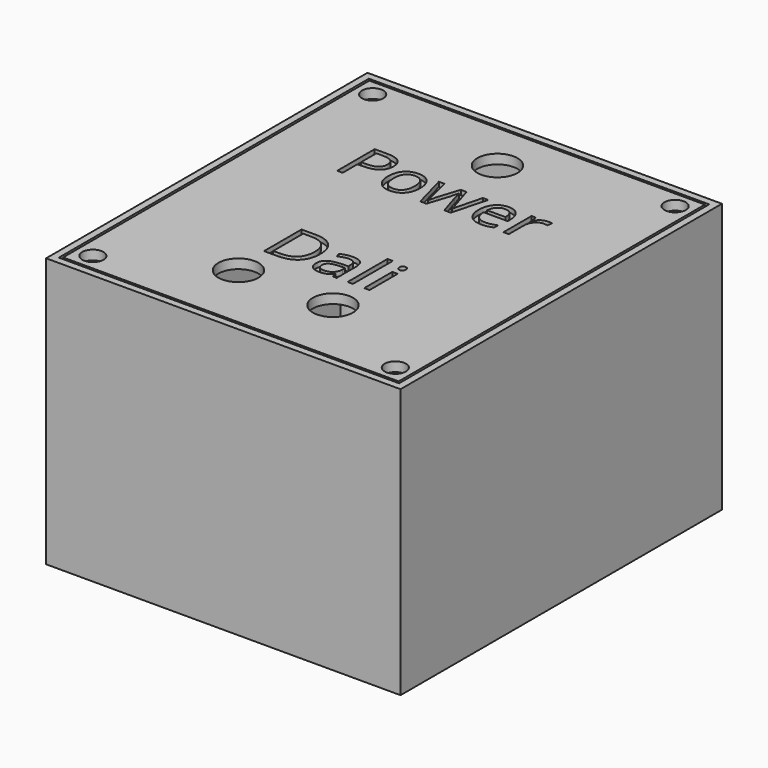
from build123d import *

# Parameters (mm, degrees)
F0_W          = 75
F0_H          = 85
F0_W_2        = 53
F0_H_2        = 63
F0_R          = 4
F1_DEPTH      = 2
F2_DEPTH      = 57
F3_DEPTH      = 9
F4_W          = 72
F4_H          = 82
F5_DEPTH      = 2
F6_D          = 3.2
F8_D          = 3.2
F8_DEPTH      = 12
F8_TIP        = 0.9613769904
F9_W          = 71
F9_H          = 81
F10_DEPTH     = 2
F11_D         = 4.5
F11_DEPTH     = 12
F11_TIP       = 1.3519363928
F13_D         = 8.5
F12_TEXT_SIZE = 13.8888888889
F14_DEPTH     = 1


# Not quite as in the source:
# - Text() gives the source's letters only with a copy of the font that has no kerning and outlines rounded to 1/6400 em; it was checked with that copy


with BuildPart() as f1:
    # F0 (on Top) → F1 (new body)
    with BuildSketch(Plane.XY):
        Rectangle(F0_W, F0_H)
        with BuildLine():
            ThreePointArc((-34, 31), (-28.3431457505, 33.3431457505), (-26, 39))
            Line((-26, 39), (26, 39))
            ThreePointArc((26, 39), (28.3431457505, 33.3431457505), (34, 31))
            Line((34, 31), (34, -31))
            ThreePointArc((34, -31), (28.3431457505, -33.3431457505), (26, -39))
            Line((26, -39), (-26, -39))
            ThreePointArc((-26, -39), (-28.3431457505, -33.3431457505), (-34, -31))
            Line((-34, -31), (-34, 31))
        make_face(mode=Mode.SUBTRACT)
        with BuildLine():
            Line((26, 39), (-26, 39))
            ThreePointArc((-26, 39), (-28.3431457505, 33.3431457505), (-34, 31))
            Line((-34, 31), (-34, -31))
            ThreePointArc((-34, -31), (-28.3431457505, -33.3431457505), (-26, -39))
            Line((-26, -39), (26, -39))
            ThreePointArc((26, -39), (28.3431457505, -33.3431457505), (34, -31))
            Line((34, -31), (34, 31))
            ThreePointArc((34, 31), (28.3431457505, 33.3431457505), (26, 39))
        make_face()
        Rectangle(F0_W_2, F0_H_2, mode=Mode.SUBTRACT)
        Rectangle(F0_W_2, F0_H_2)
        with Locations((-21.5, -26.5)):
            Circle(F0_R, mode=Mode.SUBTRACT)
        with Locations((21.5, -26.5)):
            Circle(F0_R, mode=Mode.SUBTRACT)
        with Locations((-21.5, 26.5)):
            Circle(F0_R, mode=Mode.SUBTRACT)
        with Locations((21.5, 26.5)):
            Circle(F0_R, mode=Mode.SUBTRACT)
        with Locations((-21.5, 26.5)):
            Circle(F0_R)
        with Locations((21.5, 26.5)):
            Circle(F0_R)
        with Locations((21.5, -26.5)):
            Circle(F0_R)
        with Locations((-21.5, -26.5)):
            Circle(F0_R)
    extrude(amount=F1_DEPTH)

    # F0 (on Top) → F2 (join)
    with BuildSketch(Plane.XY):
        Rectangle(F0_W, F0_H)
        with BuildLine():
            ThreePointArc((-34, 31), (-28.3431457505, 33.3431457505), (-26, 39))
            Line((-26, 39), (26, 39))
            ThreePointArc((26, 39), (28.3431457505, 33.3431457505), (34, 31))
            Line((34, 31), (34, -31))
            ThreePointArc((34, -31), (28.3431457505, -33.3431457505), (26, -39))
            Line((26, -39), (-26, -39))
            ThreePointArc((-26, -39), (-28.3431457505, -33.3431457505), (-34, -31))
            Line((-34, -31), (-34, 31))
        make_face(mode=Mode.SUBTRACT)
    extrude(amount=F2_DEPTH)

    # F0 (on Top) → F3 (join)
    with BuildSketch(Plane.XY):
        with Locations((-21.5, -26.5)):
            Circle(F0_R)
        with Locations((21.5, -26.5)):
            Circle(F0_R)
        with Locations((21.5, 26.5)):
            Circle(F0_R)
        with Locations((-21.5, 26.5)):
            Circle(F0_R)
    extrude(amount=F3_DEPTH)

    # F4 (on face) → F5 (cut)
    with BuildSketch(Plane.XY.offset(57)):
        Rectangle(F4_W, F4_H)
        with BuildLine():
            Line((26, -39), (-26, -39))
            ThreePointArc((-26, -39), (-28.3431457505, -33.3431457505), (-34, -31))
            Line((-34, -31), (-34, 31))
            ThreePointArc((-34, 31), (-28.3431457505, 33.3431457505), (-26, 39))
            Line((-26, 39), (26, 39))
            ThreePointArc((26, 39), (28.3431457505, 33.3431457505), (34, 31))
            Line((34, 31), (34, -31))
            ThreePointArc((34, -31), (28.3431457505, -33.3431457505), (26, -39))
        make_face(mode=Mode.SUBTRACT)
    extrude(amount=-F5_DEPTH, mode=Mode.SUBTRACT)

    # F6 (through all)
    with Locations(Plane(origin=(0, 0, 0), x_dir=(1, 0, 0), z_dir=(0, 0, -1))):
        with Locations((-21.5, -26.5), (21.5, -26.5), (-21.5, 26.5), (21.5, 26.5)):
            Hole(F6_D / 2)

    # F8
    with Locations(Plane.XY.offset(55)):
        with Locations((-32, -37), (-32, 37), (32, 37), (32, -37)):
            Hole(F8_D / 2, depth=F8_DEPTH)
            with Locations((0, 0, -(F8_DEPTH + F8_TIP / 2))):  # 118° drill point
                Cone(0, F8_D / 2, F8_TIP, mode=Mode.SUBTRACT)


with BuildPart() as f10:
    # F9 (on face) → F10 (new body)
    with BuildSketch(Plane.XY.offset(57)):
        Rectangle(F9_W, F9_H)
    extrude(amount=-F10_DEPTH)

    # F11
    with Locations(Plane.XY.offset(57)):
        with Locations((-32, 37), (32, 37), (32, -37), (-32, -37)):
            Hole(F11_D / 2, depth=F11_DEPTH)
            with Locations((0, 0, -(F11_DEPTH + F11_TIP / 2))):  # 118° drill point
                Cone(0, F11_D / 2, F11_TIP, mode=Mode.SUBTRACT)

    # F13 (through all)
    with Locations(Plane.XY.offset(57)):
        with Locations((0, 30), (-10, -26), (10, -26)):
            Hole(F13_D / 2)

    # F12 (on face) → F14 (cut)
    with BuildSketch(Plane.XY.offset(57)):
        with Locations((-20.8604600694, 12)):
            Text('Power', F12_TEXT_SIZE, font='Open Sans', text_align=(TextAlign.LEFT, TextAlign.BOTTOM))
        with Locations((-12.3459201389, -18)):
            Text('Dali', F12_TEXT_SIZE, font='Open Sans', text_align=(TextAlign.LEFT, TextAlign.BOTTOM))
    extrude(amount=-F14_DEPTH, mode=Mode.SUBTRACT)


solid = Compound([f1.part, f10.part])
